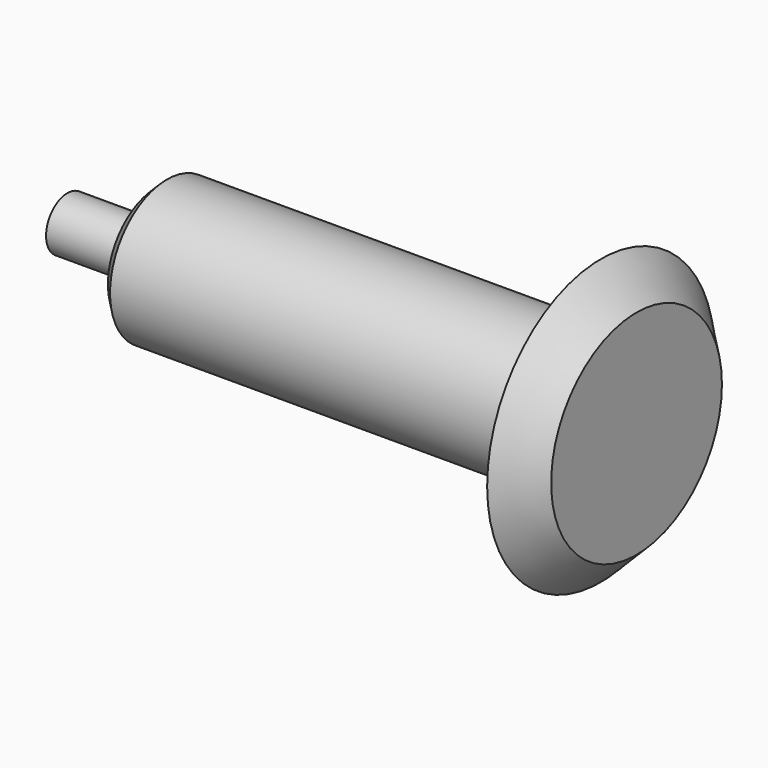
from build123d import *

# Parameters (mm, degrees)
F0_W    = 25
F0_H    = 7.5
F2_SIZE = 3
F3_SIZE = 9.99999
F4_SIZE = 9.99999


# Not quite as in the source:
# - a fillet or chamfer is up to 0.001 mm smaller than in the source, because OpenCascade refuses the exact size


with BuildPart() as f1:
    # F0 (on Top) → F1 (revolve)
    with BuildSketch(Plane.XY):
        with Locations((-54.3140277267, 3.75)):
            Rectangle(F0_W, F0_H)
        Polygon((-41.8140277267, 7.5), (-41.8140277267, 0), (73.1859722733, 0), (73.1859722733, 20), (-41.8140277267, 20), align=None)
        Polygon((73.1859722733, 20), (73.1859722733, 0), (83.1859722733, 0), (83.1859722733, 30), (73.1859722733, 30), align=None)
        Polygon((83.1859722733, 30), (83.1859722733, 0), (93.1859722733, 0), (93.1859722733, 40), (83.1859722733, 40), align=None)
    revolve(axis=Axis((15.6859722733, 0, 0), (1, 0, 0)))

    # F2
    f2_edges = [f1.edges().sort_by_distance(p)[0] for p in [
        (-41.814028, -20, 0),
    ]]
    chamfer(f2_edges, length=F2_SIZE)

    # F3 (size 10 in the source; OpenCascade refuses exactly that, so slightly less here)
    f3_edges = [f1.edges().sort_by_distance(p)[0] for p in [
        (73.185972, -30, 0),
    ]]
    chamfer(f3_edges, length=F3_SIZE)

    # F4 (size 10 in the source; OpenCascade refuses exactly that, so slightly less here)
    f4_edges = [f1.edges().sort_by_distance(p)[0] for p in [
        (93.185972, -40, 0),
    ]]
    chamfer(f4_edges, length=F4_SIZE)


solid = f1.part
